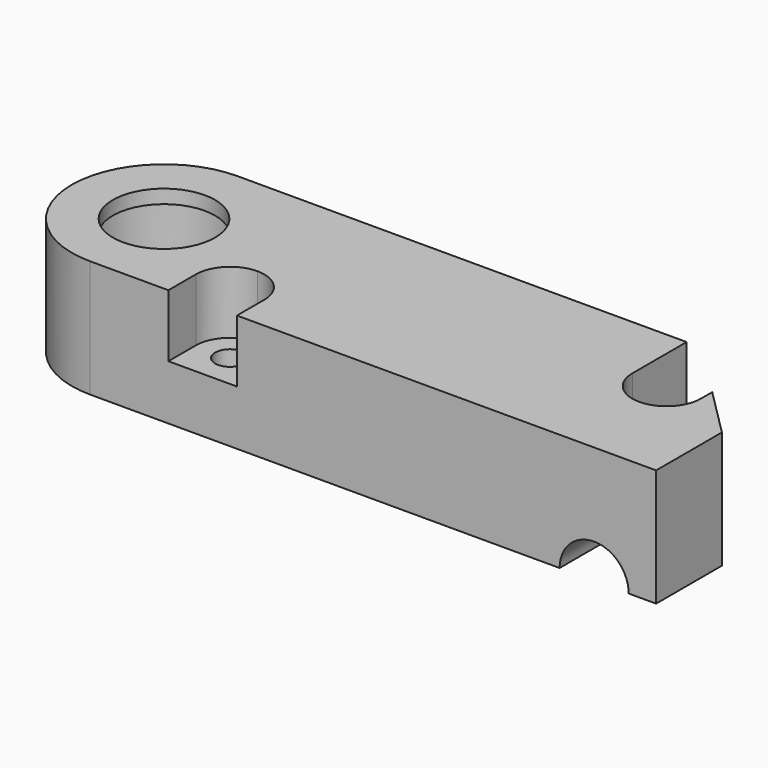
from build123d import *

# Parameters (mm, degrees)
F0_R     = 1.7272
F0_R_2   = 5.9124977
F1_DEPTH = 1.5875
F2_R     = 1.7272
F2_R_2   = 7.5
F3_DEPTH = 12
F5_DEPTH = 6.35
F6_R     = 10.674988
F7_W     = 7.9375
F7_H     = 7.9375
F8_DEPTH = 7.2375014
F9_R     = 3.96874


# Not quite as in the source:
# - a fillet or chamfer is up to 0.001 mm smaller than in the source, because OpenCascade refuses the exact size


with BuildPart() as f1:
    # F0 (on Top) → F1 (new body)
    with BuildSketch(Plane.XY):
        Polygon((64.3750046, 0), (0, 0), (0, -21.3499954), (76.2, -21.3499954), (76.2, -11.8249954), align=None)
        with Locations((23.692892633, -17.3812454)):
            Circle(F0_R, mode=Mode.SUBTRACT)
        with Locations((10.6749977, -10.6749977)):
            Circle(F0_R_2, mode=Mode.SUBTRACT)
        with Locations((66.6185899243, -7.8562454)):
            Circle(F0_R, mode=Mode.SUBTRACT)
    extrude(amount=F1_DEPTH)

    # F2 (on face) → F3 (join)
    with BuildSketch(Plane(origin=(0, 0, 0), x_dir=(1, 0, 0), z_dir=(0, 0, -1))):
        Polygon((0, 0), (64.3750046, 0), (76.2, 11.8249954), (76.2, 21.3499954), (0, 21.3499954), align=None)
        with Locations((66.6185899243, 7.8562454)):
            Circle(F2_R, mode=Mode.SUBTRACT)
        with Locations((10.6749977, 10.6749977)):
            Circle(F2_R_2, mode=Mode.SUBTRACT)
        with Locations((23.692892633, 17.3812454)):
            Circle(F2_R, mode=Mode.SUBTRACT)
    extrude(amount=F3_DEPTH)

    # F4 (on face) → F5 (cut)
    with BuildSketch(Plane.XZ.offset(21.3499954)):
        with BuildLine():
            Line((65.025, -12), (73.025, -12))
            ThreePointArc((73.025, -12), (69.025, -8), (65.025, -12))
        make_face()
    extrude(amount=-F5_DEPTH, mode=Mode.SUBTRACT)

    # F6 (radius 10.6749977 in the source; OpenCascade refuses exactly that, so slightly less here)
    f6_edges = [f1.edges().sort_by_distance(p)[0] for p in [
        (0, -21.349995, -5.20625),
        (0, 0, -5.20625),
    ]]
    fillet(f6_edges, radius=F6_R)

    # F7 (on face) → F8 (cut)
    with BuildSketch(Plane.XY.offset(1.5875)):
        with Locations((23.692892633, -17.3812454)):
            Rectangle(F7_W, F7_H)
        Polygon((64.3750046, 0), (62.6498399243, 0), (62.6498399243, -11.8249954), (70.5873399243, -11.8249954), (70.5873399243, -6.2123353243), align=None)
    extrude(amount=-F8_DEPTH, mode=Mode.SUBTRACT)

    # F9 (radius 3.96875 in the source; OpenCascade refuses exactly that, so slightly less here)
    f9_edges = [f1.edges().sort_by_distance(p)[0] for p in [
        (27.661643, -13.412495, -2.031251),
        (19.724143, -13.412495, -2.031251),
        (62.64984, -11.824995, -2.031251),
        (70.58734, -11.824995, -2.031251),
    ]]
    fillet(f9_edges, radius=F9_R)


solid = f1.part
